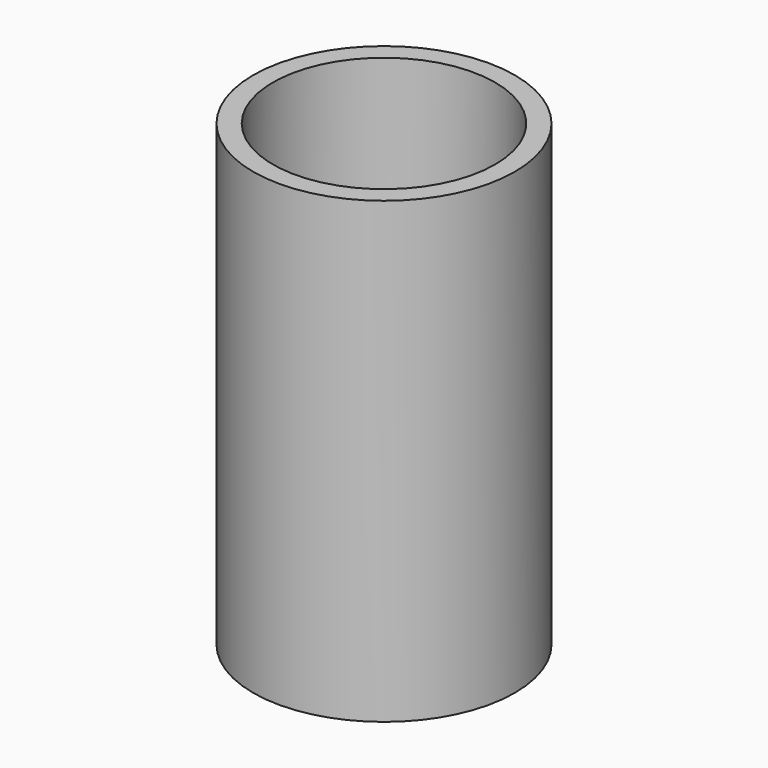
from build123d import *

# Parameters (mm, degrees)
F0_R     = 27.1625137683
F0_R_2   = 23.071077157
F1_DEPTH = 95.25
F0_R_3   = 16.1487861192
F2_DEPTH = 6
F0_R_4   = 7.8109444868
F3_DEPTH = 1.25
F4_DEPTH = 5.25


# Not quite as in the source:
# - a fillet or chamfer that OpenCascade refuses, or shapes differently, is made with other operations: its cross-section is extruded or revolved along the edge and cut away or added


with BuildPart() as f1:
    # F0 (on Top) → F1 (new body)
    with BuildSketch(Plane.XY):
        Circle(F0_R)
        Circle(F0_R_2, mode=Mode.SUBTRACT)
    extrude(amount=F1_DEPTH)

    # F0 (on Top) → F2 (join)
    with BuildSketch(Plane.XY):
        Circle(F0_R_2)
        Circle(F0_R_3, mode=Mode.SUBTRACT)
    extrude(amount=F2_DEPTH)

    # F5: fillet of radius 2 on 1 edges, made by hand

    # F5_s1 → F5_t2 (revolve, cut)
    with BuildSketch(Plane.XZ):
        with BuildLine():
            ThreePointArc((18.1497518046, -0.0004), (16.7345725568, 0.5857864376), (16.1483861192, 2.0009656854))
            Line((16.1483861192, 2.0009656854), (15.9482495506, 2.0009656854))
            ThreePointArc((15.9482495506, 2.0009656854), (15.9486495506, 1.0004828427), (15.9486495506, 0))
            Line((15.9486495506, 0), (16.1487861192, -0.2001365685))
            ThreePointArc((16.1487861192, -0.2001365685), (17.1492689619, -0.2001365685), (18.1497518046, -0.2005365685))
            Line((18.1497518046, -0.2005365685), (18.1497518046, -0.0004))
        make_face()
    revolve(axis=Axis((0, 0, 0), (0, 0, 1)), mode=Mode.SUBTRACT)


with BuildPart() as f3:
    # F0 (on Top) → F3 (new body)
    with BuildSketch(Plane.XY):
        Circle(F0_R_3)
        Circle(F0_R_4, mode=Mode.SUBTRACT)
    extrude(amount=-F3_DEPTH)

    # F0 (on Top) → F4 (join)
    with BuildSketch(Plane.XY):
        Circle(F0_R_4)
    extrude(amount=-F4_DEPTH)

    # F5#2: fillet of radius 2 on 2 edges, made by hand

    # F5_2_s1 → F5_2_t2 (revolve, cut)
    with BuildSketch(Plane.XZ):
        with BuildLine():
            ThreePointArc((7.8109444868, -3.25), (7.2251580491, -4.6642135624), (5.8109444868, -5.25))
            Line((5.8109444868, -5.25), (7.8109444868, -5.25))
            Line((7.8109444868, -5.25), (7.8109444868, -3.25))
        make_face()
    revolve(axis=Axis((0, 0, -5.25), (0, 0, 1)), mode=Mode.SUBTRACT)

    # F5_2_s3 → F5_2_t4 (revolve, cut)
    with BuildSketch(Plane.XZ):
        with BuildLine():
            ThreePointArc((16.1487861192, 0), (15.4127704861, -0.9083123952), (14.2947364974, -1.25))
            Line((14.2947364974, -1.25), (16.1487861192, -1.25))
            Line((16.1487861192, -1.25), (16.1487861192, 0))
        make_face()
    revolve(axis=Axis((0, 0, -1.25), (0, 0, 1)), mode=Mode.SUBTRACT)


solid = Compound([f1.part, f3.part])
